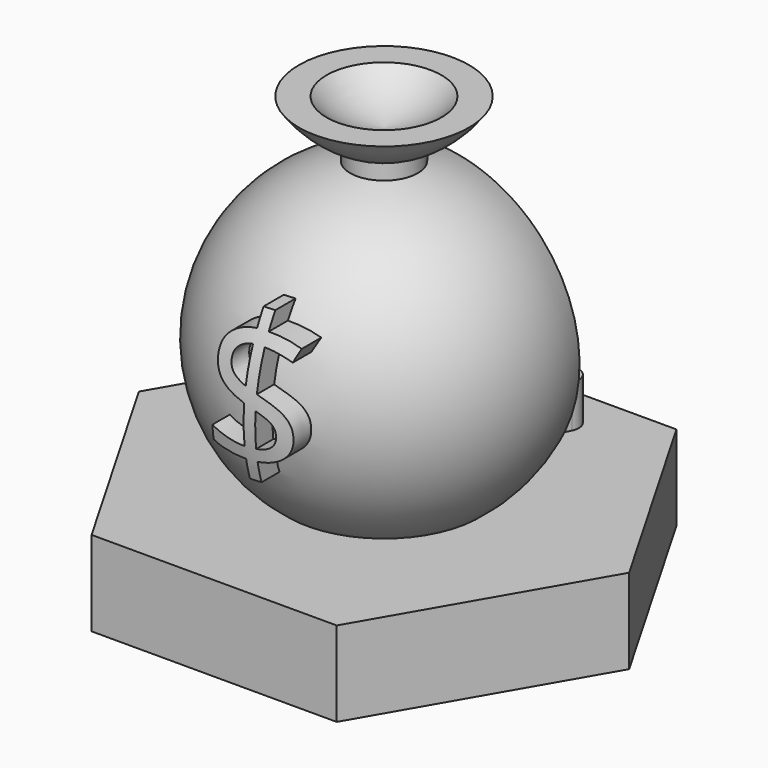
from build123d import *

# Parameters (mm, degrees)
F1_DEPTH     = 5.08
F4_TEXT_SIZE = 10.5833333333
F5_DEPTH     = 25.4
F8_W         = 18.9888755048
F8_H         = 17.78
F9_DEPTH     = 12.7
F11_DEPTH    = 2.54
F13_DEPTH    = 2.54


# Not quite as in the source:
# - Text() gives the source's letters only with a copy of the font that has no kerning and outlines rounded to 1/6400 em; it was checked with that copy


with BuildPart() as f1:
    # F0 (on Top) → F1 (new body)
    with BuildSketch(Plane.XY):
        Polygon((14.6646968374, 0), (7.3323484187, 12.7), (-7.3323484187, 12.7), (-14.6646968374, 0), (-7.3323484187, -12.7), (7.3323484187, -12.7), align=None)
    extrude(amount=F1_DEPTH)

    # F2 (on Front) → F3 (revolve)
    with BuildSketch(Plane.XZ):
        with BuildLine():
            Line((-5.715, 5.08), (0, 5.08))
            Line((0, 5.08), (0, 23.7286941882))
            ThreePointArc((0, 23.7286941882), (-1.8593893187, 24.2700707924), (-3.4321821378, 25.4))
            Line((-3.4321821378, 25.4), (-5.08, 25.4))
            ThreePointArc((-5.08, 25.4), (-3.7251362359, 23.9568888498), (-2.0204249304, 22.9508148088))
            Line((-2.0204249304, 22.9508148088), (-2.0204249304, 22.0082494649))
            ThreePointArc((-2.0204249304, 22.0082494649), (-9.3059447237, 14.7310139833), (-5.715, 5.08))
        make_face()
    revolve(axis=Axis((0, 0, 14.4043470941), (0, 0, 1)))

    # F4 (on Front) → F5 (join)
    with BuildSketch(Plane.XZ):
        with Locations((-2.4522479258, 10.16)):
            Text('$', F4_TEXT_SIZE, font='Open Sans', text_align=(TextAlign.LEFT, TextAlign.BOTTOM))
    extrude(amount=F5_DEPTH)

    # F6 (on Front) → F7 (revolve, cut)
    with BuildSketch(Plane.XZ):
        with BuildLine():
            Line((-8.1427877438, 19.7871032699), (-63.1032722388, 19.7871032699))
            ThreePointArc((-63.1032722388, 19.7871032699), (-63.4994333851, 12.4317468191), (-63.0411421216, 5.08))
            Line((-63.0411421216, 5.08), (-7.6464125575, 5.08))
            ThreePointArc((-7.6464125575, 5.08), (-10.788856899, 12.335868413), (-8.1427877438, 19.7871032699))
        make_face()
    revolve(axis=Axis((0, 0, 6.35), (0, 0, 1)), mode=Mode.SUBTRACT)

    # F8 (on Right) → F9 (cut, symmetric)
    with BuildSketch(Plane.YZ):
        with Locations((13.0956179928, 13.97)):
            Rectangle(F8_W, F8_H)
    extrude(amount=F9_DEPTH, both=True, mode=Mode.SUBTRACT)

    # F10 (on face) → F11 (join)
    with BuildSketch(Plane(origin=(0, 3.6011802404, 0), x_dir=(-1, 0, 0), z_dir=(0, 1, 0))):
        with BuildLine():
            Line((5.08, 10.2582807066), (0.6997191525, 14.0682807066))
            ThreePointArc((0.6997191525, 14.0682807066), (0, 19.05), (-0.6997191525, 14.0682807066))
            Line((-0.6997191525, 14.0682807066), (-5.08, 10.2582807066))
            ThreePointArc((-5.08, 10.2582807066), (-5.3020959391, 9.0979745195), (-4.2274533771, 8.6072807066))
            Line((-4.2274533771, 8.6072807066), (-1.905, 10.16))
            Line((-1.905, 10.16), (-1.905, 5.08))
            Line((-1.905, 5.08), (1.905, 5.08))
            Line((1.905, 5.08), (1.905, 10.16))
            Line((1.905, 10.16), (4.2274533771, 8.6072807066))
            ThreePointArc((4.2274533771, 8.6072807066), (5.3020959391, 9.0979745195), (5.08, 10.2582807066))
        make_face()
    extrude(amount=F11_DEPTH)

    # F12 (on face) → F13 (join)
    with BuildSketch(Plane.XY.offset(5.08)):
        with BuildLine():
            Line((2.0334194152, 10.3303791348), (0, 6.1411802404))
            Line((0, 6.1411802404), (1.905, 6.1411802404))
            Line((1.905, 6.1411802404), (3.5979162083, 9.5544096074))
            ThreePointArc((3.5979162083, 9.5544096074), (3.2069784988, 10.7313484388), (2.0334194152, 10.3303791348))
        make_face()
        with BuildLine():
            Line((-3.5979162083, 9.5544096074), (-1.905, 6.1411802404))
            Line((-1.905, 6.1411802404), (0, 6.1411802404))
            Line((0, 6.1411802404), (-2.0334194152, 10.3303791348))
            ThreePointArc((-2.0334194152, 10.3303791348), (-3.2069784988, 10.7313484388), (-3.5979162083, 9.5544096074))
        make_face()
    extrude(amount=F13_DEPTH)


solid = f1.part
